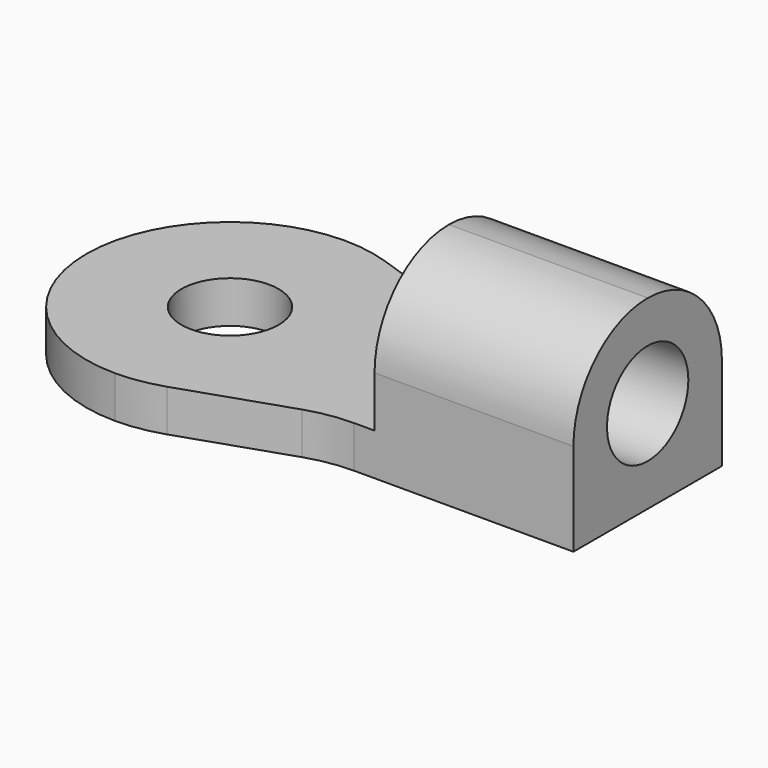
from build123d import *

# Parameters (mm, degrees)
F0_R     = 1.1
F1_DEPTH = 0.95
F2_W     = 4.5
F2_H     = 4.2
F3_DEPTH = 3.25
F4_R     = 2.09999
F5_R     = 1.15
F6_DEPTH = 25


# Not quite as in the source:
# - a fillet or chamfer is up to 0.001 mm smaller than in the source, because OpenCascade refuses the exact size


with BuildPart() as f1:
    # F0 (on Top) → F1 (new body)
    with BuildSketch(Plane.XY):
        with BuildLine():
            Line((7.7320977576, 1.15), (12.7, 1.15))
            Line((12.7, 1.15), (12.7, 5.35))
            Line((12.7, 5.35), (7.7320977576, 5.35))
            ThreePointArc((7.7320977576, 5.35), (7.2069912058, 5.3927015871), (6.6956833513, 5.5196842405))
            Line((6.6956833513, 5.5196842405), (4.2864144063, 6.3303157595))
            ThreePointArc((4.2864144063, 6.3303157595), (3.7751065518, 6.4572984129), (3.25, 6.5))
            ThreePointArc((3.25, 6.5), (0.9519029611, 5.5480970389), (0, 3.25))
            ThreePointArc((0, 3.25), (0.9519029611, 0.9519029611), (3.25, 0))
            ThreePointArc((3.25, 0), (3.7751065518, 0.0427015871), (4.2864144063, 0.1696842405))
            Line((4.2864144063, 0.1696842405), (6.6956833513, 0.9803157595))
            ThreePointArc((6.6956833513, 0.9803157595), (7.2069912058, 1.1072984129), (7.7320977576, 1.15))
        make_face()
        with Locations((3.25, 3.25)):
            Circle(F0_R, mode=Mode.SUBTRACT)
    extrude(amount=F1_DEPTH)

    # F2 (on face) → F3 (join)
    with BuildSketch(Plane.XY.offset(0.95)):
        with Locations((10.45, 3.25)):
            Rectangle(F2_W, F2_H)
    extrude(amount=F3_DEPTH)

    # F4 (radius 2.1 in the source; OpenCascade refuses exactly that, so slightly less here)
    f4_edges = [f1.edges().sort_by_distance(p)[0] for p in [
        (10.45, 5.35, 4.2),
        (10.45, 1.15, 4.2),
    ]]
    fillet(f4_edges, radius=F4_R)

    # F5 (on face) → F6 (cut)
    with BuildSketch(Plane.YZ.offset(12.7)):
        with Locations((3.25, 2.1)):
            Circle(F5_R)
    extrude(amount=-F6_DEPTH, mode=Mode.SUBTRACT)


solid = f1.part
